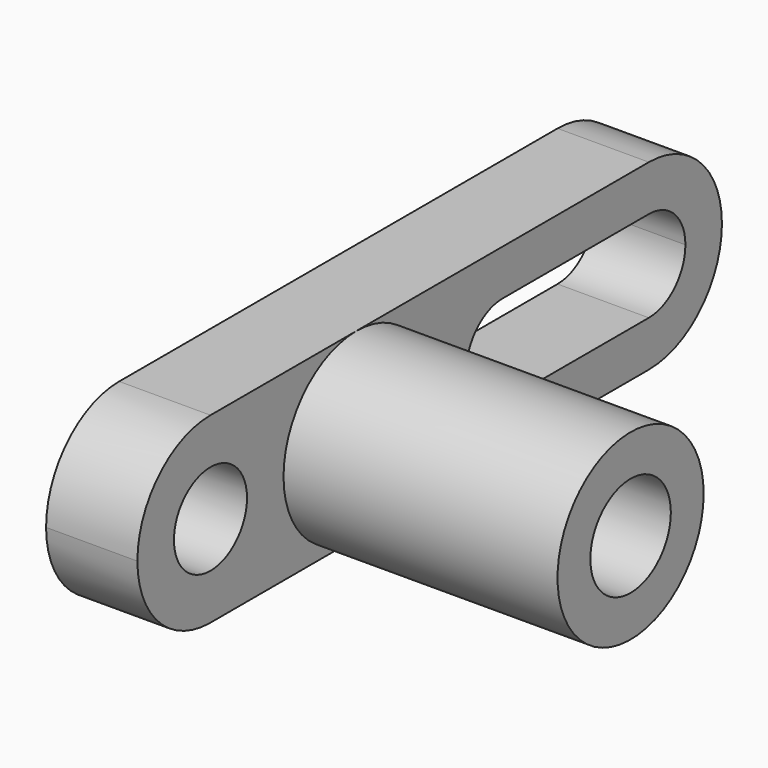
from build123d import *

# Parameters (mm, degrees)
F0_W      = 101.6
F0_H      = 25.4
F1_DEPTH  = 12.7
F3_DEPTH  = 12.7
F4_R      = 6.35
F5_DEPTH  = 12.7
F7_R      = 12.7
F8_DEPTH  = 38.1
F9_R      = 6.9951982556
F10_DEPTH = 50.8


# Not quite as in the source:
# - ends of sketch curves that miss each other by under 0.0002 mm in the source are joined


with BuildPart() as f1:
    # F0 (on Right) → F1 (new body)
    with BuildSketch(Plane.YZ):
        with Locations((50.8, 12.7)):
            Rectangle(F0_W, F0_H)
    extrude(amount=F1_DEPTH)

    # F2 (on face) → F3 (cut)
    with BuildSketch(Plane.YZ.offset(12.7)):
        with BuildLine():
            Line((0, 25.4), (0, 12.7))
            ThreePointArc((0, 12.7), (3.7197438789, 21.6802561211), (12.7, 25.4))
            Line((12.7, 25.4), (0, 25.4))
        make_face()
        with BuildLine():
            Line((0, 0), (12.7, 0))
            ThreePointArc((12.7, 0), (3.7197438789, 3.7197438789), (0, 12.7))
            Line((0, 12.7), (0, 0))
        make_face()
        with BuildLine():
            ThreePointArc((88.9, 25.4), (97.8802564546, 21.6802563035), (101.6000005159, 12.7))
            Line((101.6000005159, 12.7), (101.6, 25.4))
            Line((101.6, 25.4), (88.9, 25.4))
        make_face()
        with BuildLine():
            ThreePointArc((101.6000005159, 12.7), (97.8802568194, 3.7197440613), (88.9000010318, 0))
            Line((88.9000010318, 0), (101.6, 0))
            Line((101.6, 0), (101.6000005159, 12.7))
        make_face()
    extrude(amount=-F3_DEPTH, mode=Mode.SUBTRACT)

    # F4 (on face) → F5 (cut)
    with BuildSketch(Plane.YZ.offset(12.7)):
        with Locations((12.7, 12.7)):
            Circle(F4_R)
        with BuildLine():
            ThreePointArc((63.5000005159, 6.35), (67.9901285764, 8.2098719395), (69.8500005159, 12.7))
            ThreePointArc((69.8500005159, 12.7), (67.9901285764, 17.1901280605), (63.5000005159, 19.05))
            ThreePointArc((63.5000005159, 19.05), (57.1500005159, 12.7), (63.5000005159, 6.35))
        make_face()
        with BuildLine():
            ThreePointArc((63.5000005159, 19.05), (67.9901285764, 17.1901280605), (69.8500005159, 12.7))
            ThreePointArc((69.8500005159, 12.7), (67.9901285764, 8.2098719395), (63.5000005159, 6.35))
            Line((63.5000005159, 6.35), (88.9000005159, 6.35))
            ThreePointArc((88.9000005159, 6.35), (82.5500005159, 12.7), (88.9000005159, 19.05))
            Line((88.9000005159, 19.05), (63.5000005159, 19.05))
        make_face()
        with BuildLine():
            ThreePointArc((95.2500005159, 12.7), (93.3901285764, 17.1901280605), (88.9000005159, 19.05))
            ThreePointArc((88.9000005159, 19.05), (82.5500005159, 12.7), (88.9000005159, 6.35))
            ThreePointArc((88.9000005159, 6.35), (93.3901285764, 8.2098719395), (95.2500005159, 12.7))
        make_face()
    extrude(amount=-F5_DEPTH, mode=Mode.SUBTRACT)

    # F7 (on face) → F8 (join)
    with BuildSketch(Plane.YZ.offset(12.7)):
        with Locations((38.1, 12.7)):
            Circle(F7_R)
    extrude(amount=F8_DEPTH)

    # F9 (on face) → F10 (cut)
    with BuildSketch(Plane.YZ.offset(50.8)):
        with Locations((38.1, 12.7)):
            Circle(F9_R)
    extrude(amount=-F10_DEPTH, mode=Mode.SUBTRACT)


solid = f1.part
